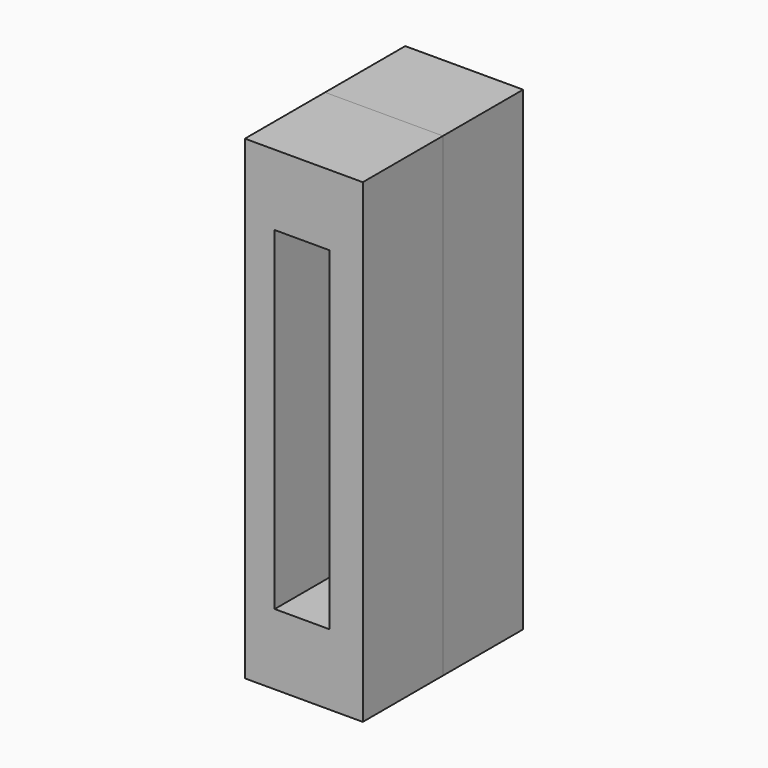
from build123d import *

# Parameters (mm, degrees)
F0_W     = 10
F0_H     = 40.3
F0_W_2   = 4.6593984449
F0_H_2   = 28.3
F1_DEPTH = 8.5
F2_DEPTH = 7


# Not quite as in the source:
# - a feature names something its author has since deleted; it is built from what else it names


with BuildPart() as f1:
    # F0 (on Front) → F1 (new body)
    with BuildSketch(Plane.XZ):
        with Locations((-25.2545091997, -60.7344553381)):
            Rectangle(F0_W, F0_H)
        with Locations((-25.3930282849, -60.7344553381)):
            Rectangle(F0_W_2, F0_H_2, mode=Mode.SUBTRACT)
        with Locations((-25.3930282849, -60.7344553381)):
            Rectangle(F0_W_2, F0_H_2)
    extrude(amount=F1_DEPTH)

    # F0 (on Front) → F2 (cut)
    with BuildSketch(Plane.XZ):
        with Locations((-25.3930282849, -60.7344553381)):
            Rectangle(F0_W_2, F0_H_2)
    extrude(amount=F2_DEPTH, mode=Mode.SUBTRACT)


with BuildPart() as f3_1:
    # F3: instance of F1
    add(f1.part.mirror(Plane(origin=(-25.2545091997, -8.5, -60.7344553381), x_dir=(1, 0, 0), z_dir=(0, -1, 0))))


solid = Compound([f1.part, f3_1.part])
